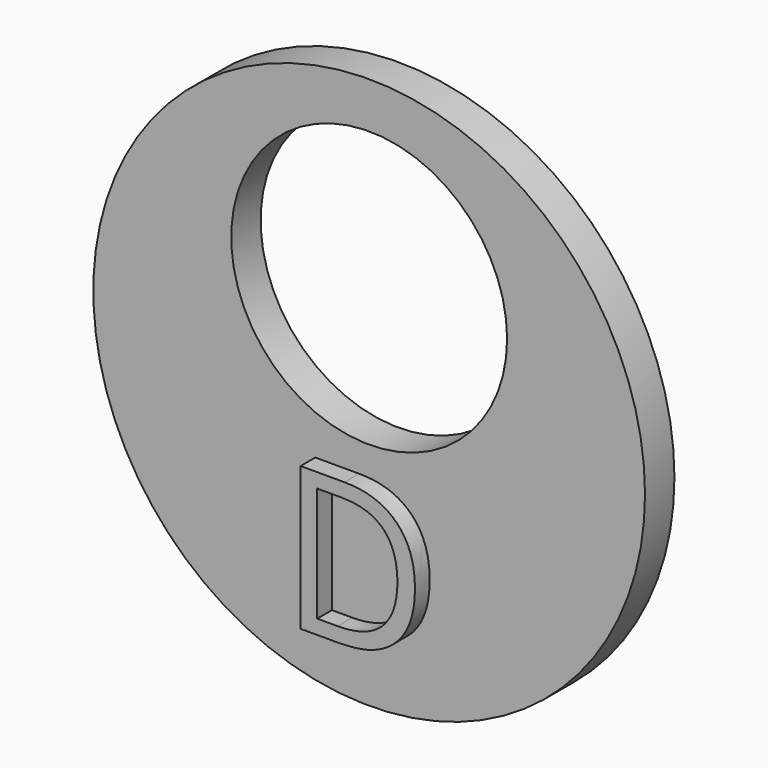
from build123d import *

# Parameters (mm, degrees)
F0_R         = 15
F0_R_2       = 7.5
F1_DEPTH     = 2
F2_TEXT_SIZE = 10.9168443497
F3_DEPTH     = 1


# Not quite as in the source:
# - Text() gives the source's letters only with a copy of the font that has no kerning and outlines rounded to 1/6400 em; it was checked with that copy


with BuildPart() as f1:
    # F0 (on Front) → F1 (new body)
    with BuildSketch(Plane.XZ):
        Circle(F0_R)
        with Locations((0, 5)):
            Circle(F0_R_2, mode=Mode.SUBTRACT)
    extrude(amount=F1_DEPTH)

    # F2 (on face) → F3 (join)
    with BuildSketch(Plane.XZ.offset(2)):
        with Locations((-4, -11.8601279318)):
            Text('D', F2_TEXT_SIZE, font='Open Sans', text_align=(TextAlign.LEFT, TextAlign.BOTTOM))
    extrude(amount=F3_DEPTH)


solid = f1.part
